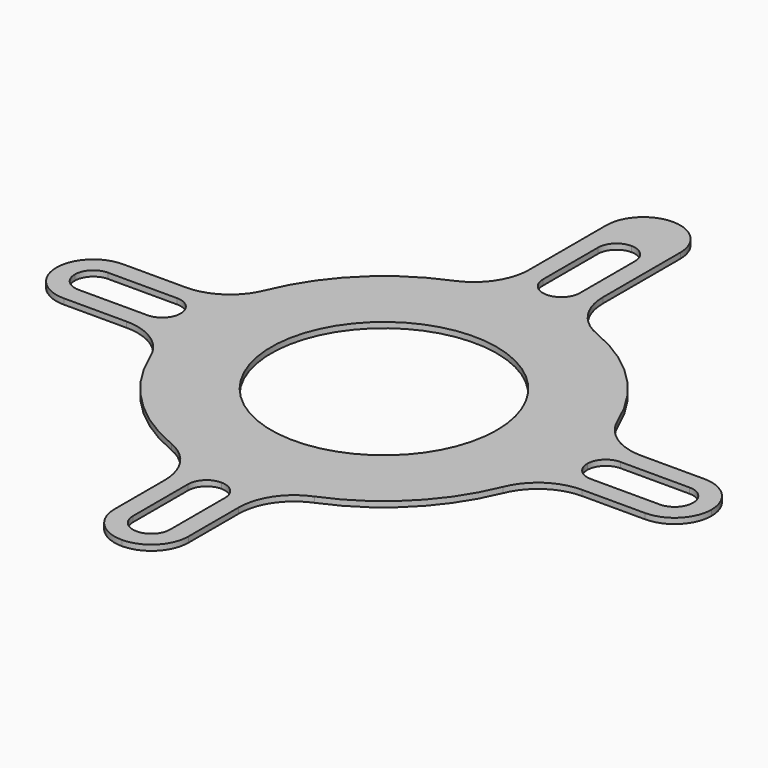
from build123d import *

# Parameters (mm, degrees)
F0_R     = 30.5
F0_W     = 5
F0_H     = 10.5
F0_W_2   = 10.5
F0_H_2   = 5
F1_DEPTH = 1.5


# Not quite as in the source:
# - a feature names something its author has since deleted; it is built from what else it names


with BuildPart() as f1:
    # F0 (on Top) → F1 (new body)
    with BuildSketch(Plane.XY):
        with BuildLine():
            ThreePointArc((-10, 61.6218305473), (-12.5584071324, 53.2428827066), (-19.3609022556, 47.7221695216))
            ThreePointArc((-19.3609022556, 47.7221695216), (-36.4159992311, 36.4159992311), (-47.7221695216, 19.3609022556))
            ThreePointArc((-47.7221695216, 19.3609022556), (-53.2428827066, 12.5584071324), (-61.6218305473, 10))
            Line((-61.6218305473, 10), (-65.6218305473, 10))
            Line((-65.6218305473, 10), (-65.6218305473, 5))
            Line((-65.6218305473, 5), (-59.986856736, 5))
            ThreePointArc((-59.986856736, 5), (-56.45132283, 3.5355339059), (-54.986856736, 0))
            ThreePointArc((-54.986856736, 0), (-56.45132283, -3.5355339059), (-59.986856736, -5))
            Line((-59.986856736, -5), (-65.6218305473, -5))
            Line((-65.6218305473, -5), (-65.6218305473, -10))
            Line((-65.6218305473, -10), (-61.6218305473, -10))
            ThreePointArc((-61.6218305473, -10), (-53.2428827066, -12.5584071324), (-47.7221695216, -19.3609022556))
            ThreePointArc((-47.7221695216, -19.3609022556), (-36.4159992311, -36.4159992311), (-19.3609022556, -47.7221695216))
            ThreePointArc((-19.3609022556, -47.7221695216), (-12.5584071324, -53.2428827066), (-10, -61.6218305473))
            Line((-10, -61.6218305473), (-10, -65.6218305473))
            Line((-10, -65.6218305473), (-5, -65.6218305473))
            Line((-5, -65.6218305473), (-5, -59.986856736))
            ThreePointArc((-5, -59.986856736), (-3.5355339059, -56.45132283), (0, -54.986856736))
            ThreePointArc((0, -54.986856736), (3.5355339059, -56.45132283), (5, -59.986856736))
            Line((5, -59.986856736), (5, -65.6218305473))
            Line((5, -65.6218305473), (10, -65.6218305473))
            Line((10, -65.6218305473), (10, -61.6218305473))
            ThreePointArc((10, -61.6218305473), (12.5584071324, -53.2428827066), (19.3609022556, -47.7221695216))
            ThreePointArc((19.3609022556, -47.7221695216), (36.4159992311, -36.4159992311), (47.7221695216, -19.3609022556))
            ThreePointArc((47.7221695216, -19.3609022556), (53.2428827066, -12.5584071324), (61.6218305473, -10))
            Line((61.6218305473, -10), (65.6218305473, -10))
            Line((65.6218305473, -10), (65.6218305473, -5))
            Line((65.6218305473, -5), (59.986856736, -5))
            ThreePointArc((59.986856736, -5), (56.45132283, -3.5355339059), (54.986856736, 0))
            ThreePointArc((54.986856736, 0), (56.45132283, 3.5355339059), (59.986856736, 5))
            Line((59.986856736, 5), (65.6218305473, 5))
            Line((65.6218305473, 5), (65.6218305473, 10))
            Line((65.6218305473, 10), (61.6218305473, 10))
            ThreePointArc((61.6218305473, 10), (53.2428827066, 12.5584071324), (47.7221695216, 19.3609022556))
            ThreePointArc((47.7221695216, 19.3609022556), (36.4159992311, 36.4159992311), (19.3609022556, 47.7221695216))
            ThreePointArc((19.3609022556, 47.7221695216), (12.5584071324, 53.2428827066), (10, 61.6218305473))
            Line((10, 61.6218305473), (10, 65.6218305473))
            Line((10, 65.6218305473), (5, 65.6218305473))
            Line((5, 65.6218305473), (5, 59.986856736))
            ThreePointArc((5, 59.986856736), (3.5355339059, 56.45132283), (0, 54.986856736))
            ThreePointArc((0, 54.986856736), (-3.5355339059, 56.45132283), (-5, 59.986856736))
            Line((-5, 59.986856736), (-5, 65.6218305473))
            Line((-5, 65.6218305473), (-10, 65.6218305473))
            Line((-10, 65.6218305473), (-10, 61.6218305473))
        make_face()
        Circle(F0_R, mode=Mode.SUBTRACT)
        with Locations((7.5, 70.8718305473)):
            Rectangle(F0_W, F0_H)
        with Locations((-7.5, 70.8718305473)):
            Rectangle(F0_W, F0_H)
        with Locations((70.8718305473, 7.5)):
            Rectangle(F0_W_2, F0_H_2)
        with Locations((70.8718305473, -7.5)):
            Rectangle(F0_W_2, F0_H_2)
        with BuildLine():
            Line((78.6218305473, 10), (76.1218305473, 10))
            Line((76.1218305473, 10), (76.1218305473, 5))
            Line((76.1218305473, 5), (78.6218305473, 5))
            ThreePointArc((78.6218305473, 5), (82.1573644532, 3.5355339059), (83.6218305473, 0))
            ThreePointArc((83.6218305473, 0), (82.1573644532, -3.5355339059), (78.6218305473, -5))
            Line((78.6218305473, -5), (76.1218305473, -5))
            Line((76.1218305473, -5), (76.1218305473, -10))
            Line((76.1218305473, -10), (78.6218305473, -10))
            ThreePointArc((78.6218305473, -10), (85.6928983592, -7.0710678119), (88.6218305473, 0))
            ThreePointArc((88.6218305473, 0), (85.6928983592, 7.0710678119), (78.6218305473, 10))
        make_face()
        with Locations((-70.8718305473, -7.5)):
            Rectangle(F0_W_2, F0_H_2)
        with Locations((-70.8718305473, 7.5)):
            Rectangle(F0_W_2, F0_H_2)
        with BuildLine():
            Line((-76.1218305473, 5), (-76.1218305473, 10))
            Line((-76.1218305473, 10), (-78.611907205, 10))
            ThreePointArc((-78.611907205, 10), (-85.6829750169, 7.0710678119), (-88.611907205, 0))
            ThreePointArc((-88.611907205, 0), (-85.6829750169, -7.0710678119), (-78.611907205, -10))
            Line((-78.611907205, -10), (-76.1218305473, -10))
            Line((-76.1218305473, -10), (-76.1218305473, -5))
            Line((-76.1218305473, -5), (-78.6218305473, -5))
            ThreePointArc((-78.6218305473, -5), (-82.1573644532, -3.5355339059), (-83.6218305473, 0))
            ThreePointArc((-83.6218305473, 0), (-82.1573644532, 3.5355339059), (-78.6218305473, 5))
            Line((-78.6218305473, 5), (-76.1218305473, 5))
        make_face()
        with Locations((-7.5, -70.8718305473)):
            Rectangle(F0_W, F0_H)
        with Locations((7.5, -70.8718305473)):
            Rectangle(F0_W, F0_H)
        with BuildLine():
            Line((-5, -76.1218305473), (-10, -76.1218305473))
            Line((-10, -76.1218305473), (-10, -78.611907205))
            ThreePointArc((-10, -78.611907205), (-7.0710678119, -85.6829750169), (0, -88.611907205))
            ThreePointArc((0, -88.611907205), (7.0710678119, -85.6829750169), (10, -78.611907205))
            Line((10, -78.611907205), (10, -76.1218305473))
            Line((10, -76.1218305473), (5, -76.1218305473))
            Line((5, -76.1218305473), (5, -78.6218305473))
            ThreePointArc((5, -78.6218305473), (3.5355339059, -82.1573644532), (0, -83.6218305473))
            ThreePointArc((0, -83.6218305473), (-3.5355339059, -82.1573644532), (-5, -78.6218305473))
            Line((-5, -78.6218305473), (-5, -76.1218305473))
        make_face()
        with BuildLine():
            Line((-10, 87.6788190633), (-10, 76.1218305473))
            Line((-10, 76.1218305473), (-5, 76.1218305473))
            Line((-5, 76.1218305473), (-5, 78.6218305473))
            ThreePointArc((-5, 78.6218305473), (-3.5355339059, 82.1573644532), (0, 83.6218305473))
            ThreePointArc((0, 83.6218305473), (3.5355339059, 82.1573644532), (5, 78.6218305473))
            Line((5, 78.6218305473), (5, 76.1218305473))
            Line((5, 76.1218305473), (10, 76.1218305473))
            Line((10, 76.1218305473), (10, 87.6788190633))
            ThreePointArc((10, 87.6788190633), (7.0710678119, 94.7498868751), (0, 97.6788190633))
            ThreePointArc((0, 97.6788190633), (-7.0710678119, 94.7498868751), (-10, 87.6788190633))
        make_face()
    extrude(amount=F1_DEPTH)


solid = f1.part
